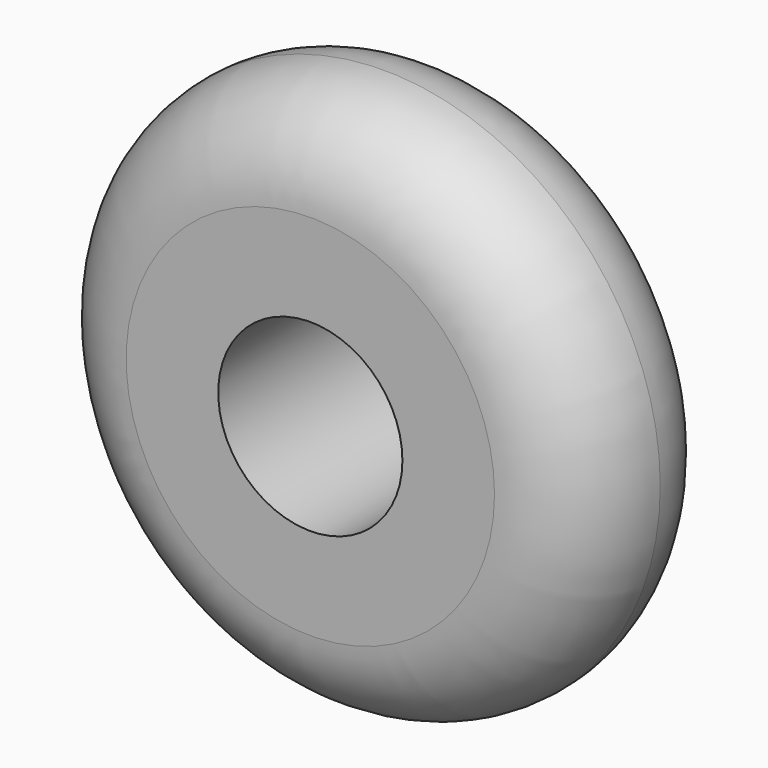
from build123d import *

# Parameters (mm, degrees)
F0_R     = 9.525
F0_R_2   = 3.175
F1_DEPTH = 6.35
F2_R     = 3.17499


# Not quite as in the source:
# - a fillet or chamfer is up to 0.001 mm smaller than in the source, because OpenCascade refuses the exact size


with BuildPart() as f1:
    # F0 (on Front) → F1 (new body)
    with BuildSketch(Plane.XZ):
        with Locations((-29.4404756278, 24.1331793368)):
            Circle(F0_R)
        with Locations((-29.4404756278, 24.1331793368)):
            Circle(F0_R_2, mode=Mode.SUBTRACT)
    extrude(amount=F1_DEPTH)

    # F2 (radius 3.175 in the source; OpenCascade refuses exactly that, so slightly less here)
    f2_edges = [f1.edges().sort_by_distance(p)[0] for p in [
        (-19.915476, -3.175, 24.133179),
        (-38.965476, 0, 24.133179),
        (-38.965476, -6.35, 24.133179),
    ]]
    fillet(f2_edges, radius=F2_R)


solid = f1.part
